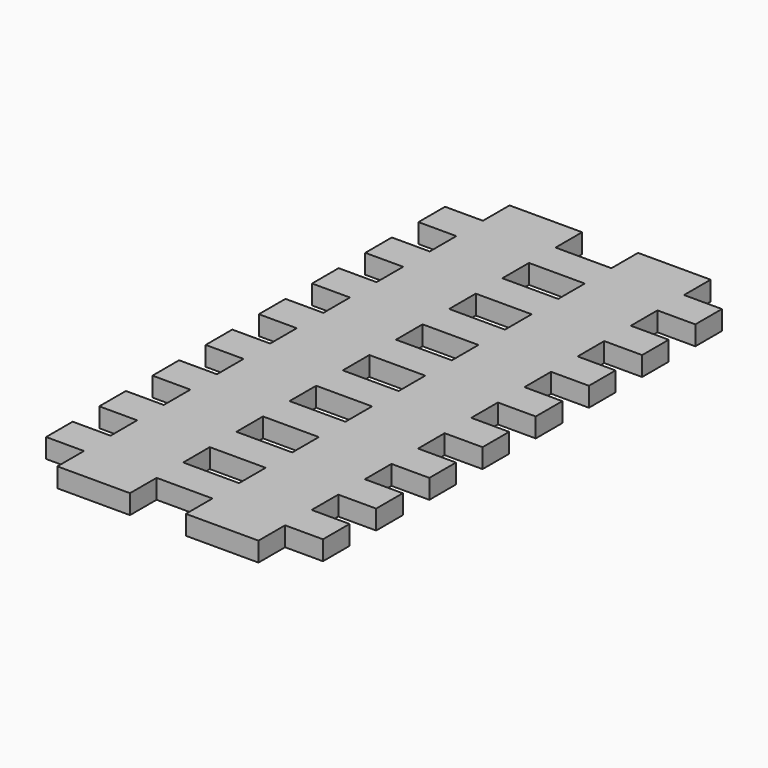
from build123d import *

# Parameters (mm, degrees)
F0_W     = 20.0313134119
F0_H     = 9.17194
F0_H_2   = 9.1719370473
F0_H_3   = 9.1719407726
F0_H_4   = 9.1719385237
F0_H_5   = 9.1719403863
F0_H_6   = 9.1719399947
F0_H_7   = 9.1719411589
F0_H_8   = 9.1719400741
F0_W_2   = 20.0313036
F0_W_3   = 15.4139306396
F0_W_4   = 10.4550179094
F0_W_5   = 10.4550202707
F0_W_6   = 10.455021
F1_DEPTH = 5.334


# Not quite as in the source:
# - ends of sketch curves that miss each other by under 0.0002 mm in the source are joined


with BuildPart() as f1:
    # F0 (on Top) → F1 (new body)
    with BuildSketch(Plane.XY):
        with Locations((-17.7226220258, 74.8951544916)):
            Rectangle(F0_W, F0_H)
        with Locations((-17.7226220258, 65.723215968)):
            Rectangle(F0_W, F0_H_2)
        with Locations((-17.7226220258, 47.3793366717)):
            Rectangle(F0_W, F0_H)
        with Locations((-17.7226220258, 56.551277058)):
            Rectangle(F0_W, F0_H_3)
        with Locations((-17.7226220258, 38.2073974099)):
            Rectangle(F0_W, F0_H_4)
        with Locations((-17.7226220258, 29.0354579549)):
            Rectangle(F0_W, F0_H_5)
        with Locations((-17.7226220258, -16.824242307)):
            Rectangle(F0_W, F0_H)
        with Locations((-17.7226220258, 1.5196376903)):
            Rectangle(F0_W, F0_H_6)
        with Locations((-17.7226220258, -35.1681232728)):
            Rectangle(F0_W, F0_H_7)
        with Locations((-17.7226220258, 10.6915776877)):
            Rectangle(F0_W, F0_H)
        with Locations((-17.7226220258, -7.652302307)):
            Rectangle(F0_W, F0_H)
        with Locations((-17.7226220258, -53.5120038522)):
            Rectangle(F0_W, F0_H)
        with Locations((-17.7226220258, -25.9961825002)):
            Rectangle(F0_W, F0_H_5)
        with Locations((-17.7226220258, -44.3400638522)):
            Rectangle(F0_W, F0_H)
        with Locations((-17.7226220258, -62.6839438522)):
            Rectangle(F0_W, F0_H)
        with Locations((-17.7226220258, 19.8635177247)):
            Rectangle(F0_W, F0_H_8)
        with Locations((17.7226171198, 29.0354579549)):
            Rectangle(F0_W_2, F0_H_5)
        with Locations((17.7226171198, 47.3793366717)):
            Rectangle(F0_W_2, F0_H)
        with Locations((17.7226171198, -62.6839438522)):
            Rectangle(F0_W_2, F0_H)
        with Locations((17.7226171198, 19.8635177247)):
            Rectangle(F0_W_2, F0_H_8)
        with Locations((17.7226171198, -53.5120038522)):
            Rectangle(F0_W_2, F0_H)
        with Locations((17.7226171198, -25.9961825002)):
            Rectangle(F0_W_2, F0_H_5)
        with Locations((17.7226171198, -7.652302307)):
            Rectangle(F0_W_2, F0_H)
        with Locations((17.7226171198, 38.2073974099)):
            Rectangle(F0_W_2, F0_H_4)
        with Locations((17.7226171198, -35.1681232728)):
            Rectangle(F0_W_2, F0_H_7)
        with Locations((17.7226171198, 10.6915776877)):
            Rectangle(F0_W_2, F0_H)
        with Locations((17.7226171198, -44.3400638522)):
            Rectangle(F0_W_2, F0_H)
        with Locations((17.7226171198, 65.723215968)):
            Rectangle(F0_W_2, F0_H_2)
        with Locations((17.7226171198, 74.8951544916)):
            Rectangle(F0_W_2, F0_H)
        with Locations((17.7226171198, 56.551277058)):
            Rectangle(F0_W_2, F0_H_3)
        with Locations((17.7226171198, -16.824242307)):
            Rectangle(F0_W_2, F0_H)
        with Locations((17.7226171198, 1.5196376903)):
            Rectangle(F0_W_2, F0_H_6)
        Polygon((27.7382689198, 70.3091844916), (27.7382689198, 61.1372474443), (38.1932891905, 61.1372474443), (38.1932891905, 70.3091878306), align=None)
        with Locations((0, 65.723215968)):
            Rectangle(F0_W_3, F0_H_2)
        with Locations((-32.9657876864, 65.723215968)):
            Rectangle(F0_W_4, F0_H_2)
        with Locations((-32.9657876864, 47.3793366717)):
            Rectangle(F0_W_4, F0_H)
        with Locations((0, 47.3793366717)):
            Rectangle(F0_W_3, F0_H)
        with Locations((32.9657790552, 47.3793366717)):
            Rectangle(F0_W_5, F0_H)
        with Locations((32.9657790552, 29.0354579549)):
            Rectangle(F0_W_5, F0_H_5)
        with Locations((0, 29.0354579549)):
            Rectangle(F0_W_3, F0_H_5)
        with Locations((-32.9657876864, 29.0354579549)):
            Rectangle(F0_W_4, F0_H_5)
        with Locations((-32.9657876864, 10.6915776877)):
            Rectangle(F0_W_4, F0_H)
        with Locations((32.9657790552, 10.6915776877)):
            Rectangle(F0_W_5, F0_H)
        with Locations((32.9657790552, -7.652302307)):
            Rectangle(F0_W_5, F0_H)
        with Locations((-32.9657876864, -7.652302307)):
            Rectangle(F0_W_4, F0_H)
        with Locations((-32.9657876864, -25.9961825002)):
            Rectangle(F0_W_4, F0_H_5)
        with Locations((0, 10.6915776877)):
            Rectangle(F0_W_3, F0_H)
        with Locations((0, -7.652302307)):
            Rectangle(F0_W_3, F0_H)
        with Locations((0, -25.9961825002)):
            Rectangle(F0_W_3, F0_H_5)
        with Locations((0, -44.3400638522)):
            Rectangle(F0_W_3, F0_H)
        with Locations((32.9657794198, -25.9961825002)):
            Rectangle(F0_W_6, F0_H_5)
        with Locations((32.9657794198, -44.3400638522)):
            Rectangle(F0_W_6, F0_H)
        with Locations((-32.9657876864, -44.3400638522)):
            Rectangle(F0_W_4, F0_H)
        with Locations((-32.9657876864, -62.6839438522)):
            Rectangle(F0_W_4, F0_H)
        with Locations((0, -62.6839438522)):
            Rectangle(F0_W_3, F0_H)
        with Locations((32.9657794198, -62.6839438522)):
            Rectangle(F0_W_6, F0_H)
        with Locations((-17.7226220258, -71.8558840454)):
            Rectangle(F0_W, F0_H_5)
        with Locations((17.7226171198, -71.8558840454)):
            Rectangle(F0_W_2, F0_H_5)
    extrude(amount=F1_DEPTH)


solid = f1.part
